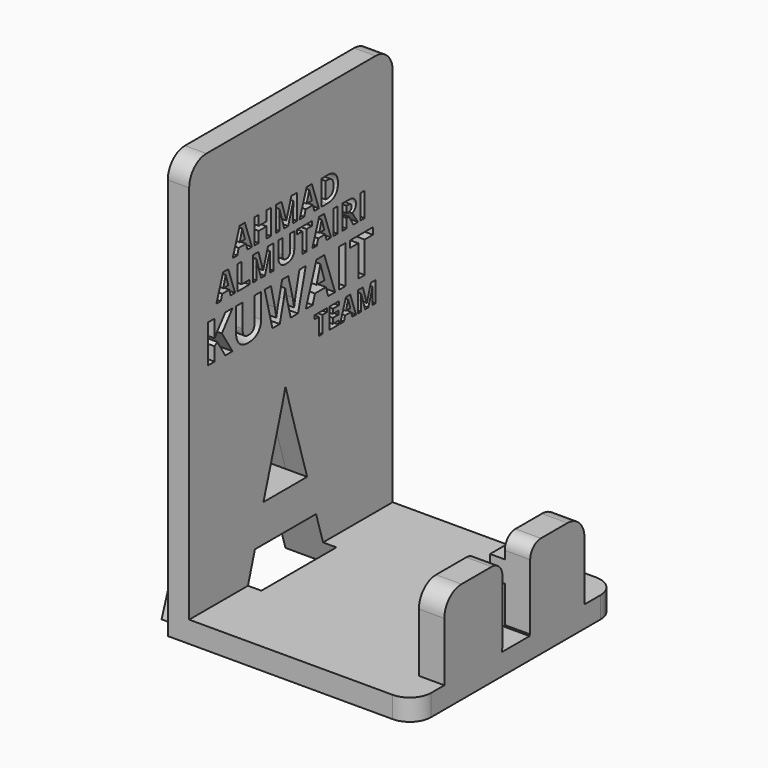
from build123d import *

# Parameters (mm, degrees)
F0_W          = 92
F0_H          = 95
F1_DEPTH      = 8
F2_W          = 8
F2_H          = 95
F3_DEPTH      = 150
F4_W          = 9.502086699
F4_H          = 65.4331929982
F5_DEPTH      = 30
F6_TEXT_SIZE  = 109.7222222222
F7_DEPTH      = 8
F8_DEPTH      = 13
F9_W          = 92.7244275808
F9_H          = 12.8235910088
F10_DEPTH     = 8
F11_T1_DEPTH  = 9.502086699
F11_T3_DEPTH  = 49.502086699
F11_T5_DEPTH  = 48
F11_T7_DEPTH  = 48
F11_T9_DEPTH  = 22.1511570575
F11_T11_DEPTH = 22.1686230261
F13_W         = 50
F13_H         = 8
F14_DEPTH     = 15
F15_W         = 13
F15_H         = 30
F16_DEPTH     = 51
F17_R         = 5
F21_TEXT_SIZE = 12.6808004755
F18_TEXT_SIZE = 19.8418849791
F19_TEXT_SIZE = 10.7493562003
F20_TEXT_SIZE = 13.037809648
F22_DEPTH     = 25


# Not quite as in the source:
# - a fillet or chamfer that OpenCascade refuses, or shapes differently, is made with other operations: its cross-section is extruded or revolved along the edge and cut away or added
# - Text() gives the source's letters only with a copy of the font that has no kerning and outlines rounded to 1/6400 em; it was checked with that copy


with BuildPart() as f1:
    # F0 (on Top) → F1 (new body)
    with BuildSketch(Plane.XY):
        Rectangle(F0_W, F0_H)
    extrude(amount=F1_DEPTH)

    # F2 (on face) → F3 (join)
    with BuildSketch(Plane.XY.offset(8)):
        with Locations((-42, 0)):
            Rectangle(F2_W, F2_H)
    extrude(amount=F3_DEPTH)

    # F4 (on face) → F5 (join)
    with BuildSketch(Plane.XY.offset(8)):
        with Locations((41.2489566505, -0.6576199085)):
            Rectangle(F4_W, F4_H)
    extrude(amount=F5_DEPTH)

    # F6 (on face) → F7 (join)
    with BuildSketch(Plane(origin=(-46, 0, 0), x_dir=(0, -1, 0), z_dir=(-1, 0, 0))):
        with Locations((-35.3231336806, 0)):
            Text('A', F6_TEXT_SIZE, font='Open Sans', font_style=FontStyle.BOLD, text_align=(TextAlign.LEFT, TextAlign.BOTTOM))
    extrude(amount=F7_DEPTH)

    # F8 (cut): faces of the model
    f8_faces = [f1.faces().sort_by_distance(p)[0] for p in [
        (-46, -2.6092958686, 43.7110655024),
        (-46, -2.5310329861, 8.8111101838),
    ]]
    extrude(f8_faces, amount=-F8_DEPTH, mode=Mode.SUBTRACT)

    # F9 (on face) → F10 (cut)
    with BuildSketch(Plane.XY.offset(8)):
        Rectangle(F9_W, F9_H)
    extrude(amount=F10_DEPTH, mode=Mode.SUBTRACT)

    # F11: fillet of radius 8 on 10 edges, made by hand

    # F11_s2 → F11_t1 (join)
    with BuildSketch(Plane.YZ.offset(36.497913301)):
        with BuildLine():
            ThreePointArc((1.5882044956, 16), (-4.0686497539, 13.6568542495), (-6.4117955044, 8))
            Line((-6.4117955044, 8), (-6.4117955044, 16))
            Line((-6.4117955044, 16), (1.5882044956, 16))
        make_face()
        with BuildLine():
            ThreePointArc((6.4117955044, 8), (4.0686497539, 13.6568542495), (-1.5882044956, 16))
            Line((-1.5882044956, 16), (6.4117955044, 16))
            Line((6.4117955044, 16), (6.4117955044, 8))
        make_face()
    extrude(amount=F11_T1_DEPTH)

    # F11_s4 → F11_t3 (cut)
    with BuildSketch(Plane.YZ.offset(16.497913301)):
        with BuildLine():
            ThreePointArc((-33.3742164075, 30), (-31.031070657, 35.6568542495), (-25.3742164075, 38))
            Line((-25.3742164075, 38), (-33.3742164075, 38))
            Line((-33.3742164075, 38), (-33.3742164075, 30))
        make_face()
        with BuildLine():
            ThreePointArc((24.0589765906, 38), (29.7158308401, 35.6568542495), (32.0589765906, 30))
            Line((32.0589765906, 30), (32.0589765906, 38))
            Line((32.0589765906, 38), (24.0589765906, 38))
        make_face()
    extrude(amount=F11_T3_DEPTH, mode=Mode.SUBTRACT)

    # F11_s6 → F11_t5 (cut)
    with BuildSketch(Plane.XY.offset(-20)):
        with BuildLine():
            ThreePointArc((38, -47.5), (43.6568542495, -45.1568542495), (46, -39.5))
            Line((46, -39.5), (46, -47.5))
            Line((46, -47.5), (38, -47.5))
        make_face()
        with BuildLine():
            ThreePointArc((38, 47.5), (43.6568542495, 45.1568542495), (46, 39.5))
            Line((46, 39.5), (46, 47.5))
            Line((46, 47.5), (38, 47.5))
        make_face()
    extrude(amount=F11_T5_DEPTH, mode=Mode.SUBTRACT)

    # F11_s8 → F11_t7 (cut)
    with BuildSketch(Plane.YZ.offset(-66)):
        with BuildLine():
            ThreePointArc((47.5, 150), (45.1568542495, 155.6568542495), (39.5, 158))
            Line((39.5, 158), (47.5, 158))
            Line((47.5, 158), (47.5, 150))
        make_face()
        with BuildLine():
            ThreePointArc((-47.5, 150), (-45.1568542495, 155.6568542495), (-39.5, 158))
            Line((-39.5, 158), (-47.5, 158))
            Line((-47.5, 158), (-47.5, 150))
        make_face()
    extrude(amount=F11_T7_DEPTH, mode=Mode.SUBTRACT)

    # F11_s10 → F11_t9 (cut)
    with BuildSketch(Plane.YZ.offset(-68.1511570575)):
        with BuildLine():
            ThreePointArc((-6.968443427, 78.6571180556), (-11.5892092127, 77.1877017625), (-14.5125178655, 73.3192489439))
            Line((-14.5125178655, 73.3192489439), (-12.62890625, 78.6571180556))
            Line((-12.62890625, 78.6571180556), (-6.968443427, 78.6571180556))
        make_face()
    extrude(amount=F11_T9_DEPTH, mode=Mode.SUBTRACT)

    # F11_s12 → F11_t11 (cut)
    with BuildSketch(Plane.YZ.offset(-68.1686230261)):
        with BuildLine():
            ThreePointArc((9.5494221686, 73.3104701901), (6.6268195719, 77.1850127038), (2.0022556507, 78.6571180556))
            Line((2.0022556507, 78.6571180556), (7.6697048611, 78.6571180556))
            Line((7.6697048611, 78.6571180556), (9.5494221686, 73.3104701901))
        make_face()
    extrude(amount=F11_T11_DEPTH, mode=Mode.SUBTRACT)

    # F13 (on face) → F14 (join)
    with BuildSketch(Plane.YZ.offset(46)):
        with Locations((-0.3742164075, 26)):
            Rectangle(F13_W, F13_H)
    extrude(amount=-F14_DEPTH)

    # F15 (on Right) → F16 (cut)
    with BuildSketch(Plane.YZ):
        with Locations((0.2138538808, 23.445661515)):
            Rectangle(F15_W, F15_H)
    extrude(amount=F16_DEPTH, mode=Mode.SUBTRACT)

    # F17
    f17_edges = [f1.edges().sort_by_distance(p)[0] for p in [
        (41.248957, -6.286146, 38),
        (41.248957, 6.713854, 38),
    ]]
    fillet(f17_edges, radius=F17_R)

    # F21 (on face) + F18 (on face) + F19 (on face) + F20 (on face) → F22 (cut)
    with BuildSketch(Plane.YZ.offset(-38)):
        with Locations((-34.8122259855, 106.7333307635)):
            Text('ALMUTAIRI', F21_TEXT_SIZE, font='Open Sans', font_style=FontStyle.BOLD, text_align=(TextAlign.LEFT, TextAlign.BOTTOM))
    with BuildSketch(Plane.YZ.offset(-38)):
        with Locations((-40.433262405, 88.0184907196)):
            Text('KUWAIT', F18_TEXT_SIZE, font='Open Sans', font_style=FontStyle.BOLD, text_align=(TextAlign.LEFT, TextAlign.BOTTOM))
    with BuildSketch(Plane.YZ.offset(-38)):
        with Locations((10.734507814, 76.6298472881)):
            Text('TEAM', F19_TEXT_SIZE, font='Open Sans', font_style=FontStyle.BOLD, text_align=(TextAlign.LEFT, TextAlign.BOTTOM))
    with BuildSketch(Plane.YZ.offset(-38)):
        with Locations((-27.1967503495, 118.6231198336)):
            Text('AHMAD', F20_TEXT_SIZE, font='Open Sans', font_style=FontStyle.BOLD, text_align=(TextAlign.LEFT, TextAlign.BOTTOM))
    extrude(amount=-F22_DEPTH, mode=Mode.SUBTRACT)


solid = f1.part
